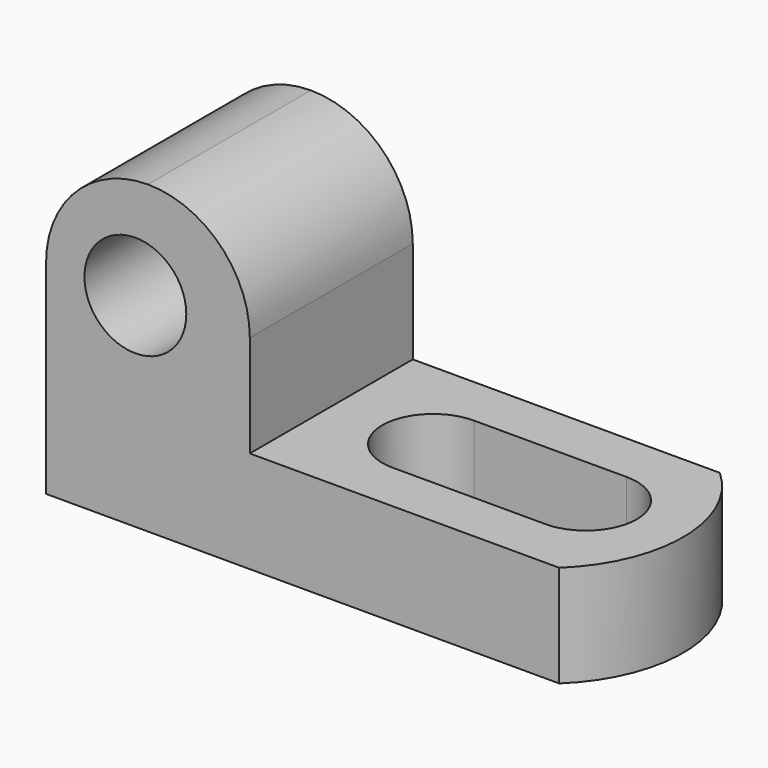
from build123d import *

# Parameters (mm, degrees)
F0_W      = 69.85
F0_H      = 38.1
F1_DEPTH  = 25.4
F2_W      = 44.45
F2_H      = 25.4
F3_DEPTH  = 25.4
F4_R      = 12.69999
F5_R      = 6.35
F6_DEPTH  = 25.4
F8_DEPTH  = 50.8
F10_DEPTH = 50.8


# Not quite as in the source:
# - a fillet or chamfer is up to 0.001 mm smaller than in the source, because OpenCascade refuses the exact size


with BuildPart() as f1:
    # F0 (on Front) → F1 (new body)
    with BuildSketch(Plane.XZ):
        with Locations((34.925, 19.05)):
            Rectangle(F0_W, F0_H)
    extrude(amount=F1_DEPTH)

    # F2 (on face) → F3 (cut)
    with BuildSketch(Plane.XZ.offset(25.4)):
        with Locations((47.625, 25.4)):
            Rectangle(F2_W, F2_H)
    extrude(amount=-F3_DEPTH, mode=Mode.SUBTRACT)

    # F4 (radius 12.7 in the source; OpenCascade refuses exactly that, so slightly less here)
    f4_edges = [f1.edges().sort_by_distance(p)[0] for p in [
        (25.4, -12.7, 38.1),
        (0, -12.7, 38.1),
    ]]
    fillet(f4_edges, radius=F4_R)

    # F5 (on face) → F6 (cut)
    with BuildSketch(Plane.XZ.offset(25.4)):
        with Locations((11.1332936212, 25.4)):
            Circle(F5_R)
    extrude(amount=-F6_DEPTH, mode=Mode.SUBTRACT)

    # F7 (on face) → F8 (cut)
    with BuildSketch(Plane.XY.offset(12.7)):
        with BuildLine():
            ThreePointArc((38.1, -19.05), (42.5901280605, -17.1901280605), (44.45, -12.7))
            ThreePointArc((44.45, -12.7), (42.5901280605, -8.2098719395), (38.1, -6.35))
            ThreePointArc((38.1, -6.35), (31.75, -12.7), (38.1, -19.05))
        make_face()
        with BuildLine():
            ThreePointArc((38.1, -6.35), (42.5901280605, -8.2098719395), (44.45, -12.7))
            ThreePointArc((44.45, -12.7), (42.5901280605, -17.1901280605), (38.1, -19.05))
            Line((38.1, -19.05), (57.15, -19.05))
            ThreePointArc((57.15, -19.05), (50.8, -12.7), (57.15, -6.35))
            Line((57.15, -6.35), (38.1, -6.35))
        make_face()
        with BuildLine():
            ThreePointArc((63.5, -12.7), (61.6401280605, -8.2098719395), (57.15, -6.35))
            ThreePointArc((57.15, -6.35), (50.8, -12.7), (57.15, -19.05))
            ThreePointArc((57.15, -19.05), (61.6401280605, -17.1901280605), (63.5, -12.7))
        make_face()
    extrude(amount=-F8_DEPTH, mode=Mode.SUBTRACT)

    # F9 (on face) → F10 (cut)
    with BuildSketch(Plane.XY.offset(12.7)):
        with BuildLine():
            ThreePointArc((63.6959075928, 0), (69.3784721841, -12.6381087117), (63.9796331525, -25.4))
            Line((63.9796331525, -25.4), (69.85, -25.4))
            Line((69.85, -25.4), (69.85, 0))
            Line((69.85, 0), (63.6959075928, 0))
        make_face()
    extrude(amount=-F10_DEPTH, mode=Mode.SUBTRACT)


solid = f1.part
